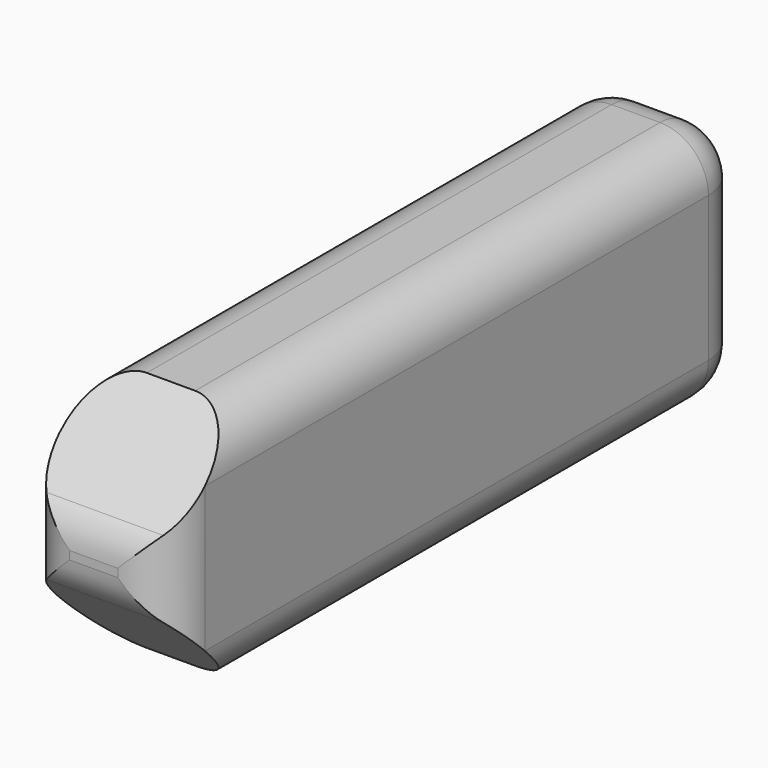
from build123d import *

# Parameters (mm, degrees)
F0_W     = 75
F0_H     = 25
F1_DEPTH = 15
F2_SIZE  = 10
F3_SIZE  = 10
F4_R     = 5
F5_R     = 5
F6_R     = 4.99999


# Not quite as in the source:
# - a fillet or chamfer is up to 0.001 mm smaller than in the source, because OpenCascade refuses the exact size


with BuildPart() as f1:
    # F0 (on Right) → F1 (new body)
    with BuildSketch(Plane.YZ):
        Rectangle(F0_W, F0_H)
    extrude(amount=F1_DEPTH)

    # F2
    f2_edges = [f1.edges().sort_by_distance(p)[0] for p in [
        (7.5, -37.5, 12.5),
    ]]
    chamfer(f2_edges, length=F2_SIZE)

    # F3
    f3_edges = [f1.edges().sort_by_distance(p)[0] for p in [
        (7.5, -37.5, -12.5),
    ]]
    chamfer(f3_edges, length=F3_SIZE)

    # F4
    f4_edges = [f1.edges().sort_by_distance(p)[0] for p in [
        (15, 5, 12.5),
        (0, 5, 12.5),
        (15, 5, -12.5),
        (0, 5, -12.5),
    ]]
    fillet(f4_edges, radius=F4_R)

    # F5
    f5_edges = [f1.edges().sort_by_distance(p)[0] for p in [
        (7.5, 37.5, -12.5),
        (1.464466, 37.5, -11.035534),
        (13.535534, 37.5, -11.035534),
        (0, 37.5, 0),
        (15, 37.5, 0),
        (1.464466, 37.5, 11.035534),
        (13.535534, 37.5, 11.035534),
        (7.5, 37.5, 12.5),
    ]]
    fillet(f5_edges, radius=F5_R)

    # F6 (radius 5 in the source; OpenCascade refuses exactly that, so slightly less here)
    f6_edges = [f1.edges().sort_by_distance(p)[0] for p in [
        (0, -37.5, 0),
        (7.5, -37.5, -2.5),
        (7.5, -37.5, 2.5),
        (15, -37.5, 0),
    ]]
    fillet(f6_edges, radius=F6_R)


solid = f1.part
